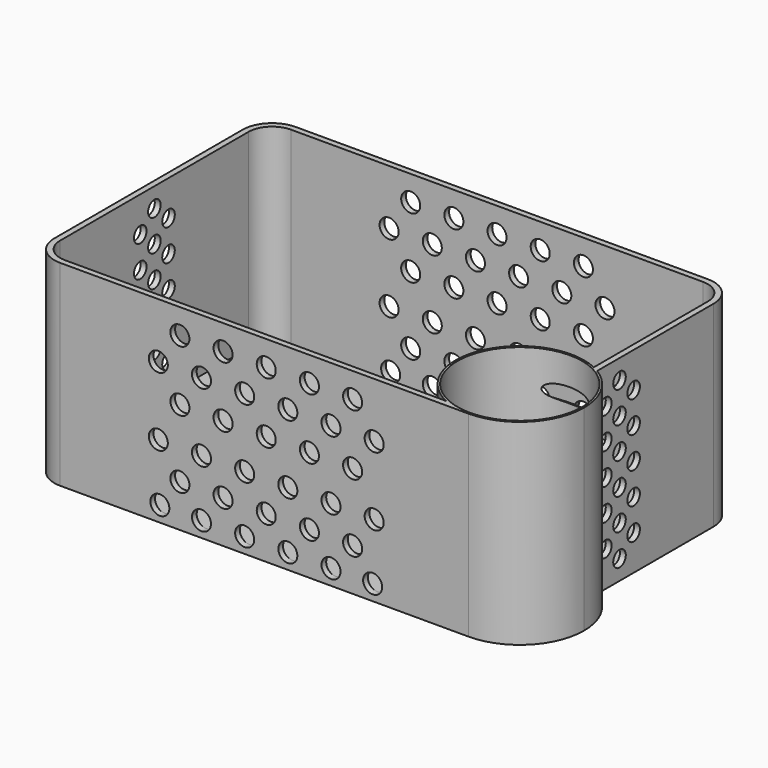
from build123d import *

# Parameters (mm, degrees)
F0_R     = 31.75
F1_DEPTH = 100
F3_DEPTH = 3
F5_D     = 9.7
F7_D     = 8


# Not quite as in the source:
# - a feature names something its author has since deleted; it is built from what else it names


with BuildPart() as f1:
    # F0 (on Top) → F1 (new body)
    with BuildSketch(Plane.XY):
        with BuildLine():
            Line((105, 75), (-105, 75))
            ThreePointArc((-105, 75), (-115.6066017178, 70.6066017178), (-120, 60))
            Line((-120, 60), (-120, -60))
            ThreePointArc((-120, -60), (-115.6066017178, -70.6066017178), (-105, -75))
            Line((-105, -75), (103, -75))
            ThreePointArc((103, -75), (95.9910771156, -74.2412097302), (89.3069360624, -72))
            Line((89.3069360624, -72), (-105, -72))
            ThreePointArc((-105, -72), (-113.4852813742, -68.4852813742), (-117, -60))
            Line((-117, -60), (-117, 60))
            ThreePointArc((-117, 60), (-113.4852813742, 68.4852813742), (-105, 72))
            Line((-105, 72), (105, 72))
            ThreePointArc((105, 72), (113.4852813742, 68.4852813742), (117, 60))
            Line((117, 60), (117, -12.6432017942))
            ThreePointArc((117, -12.6432017942), (118.5210097227, -13.4114709601), (120, -14.2578135902))
            Line((120, -14.2578135902), (120, 60))
            ThreePointArc((120, 60), (115.6066017178, 70.6066017178), (105, 75))
        make_face()
        with BuildLine():
            ThreePointArc((135.75, -42.25), (131.5421836936, -26.190540171), (120, -14.2578135902))
            ThreePointArc((120, -14.2578135902), (118.5210097227, -13.4114709601), (117, -12.6432017942))
            ThreePointArc((117, -12.6432017942), (73.3212041055, -28.4032829071), (89.3069360624, -72))
            ThreePointArc((89.3069360624, -72), (95.9910771156, -74.2412097302), (103, -75))
            ThreePointArc((103, -75), (126.1577470839, -65.4077470839), (135.75, -42.25))
        make_face()
        with Locations((103, -42.25)):
            Circle(F0_R, mode=Mode.SUBTRACT)
    extrude(amount=F1_DEPTH)

    # F2 (on Top) → F3 (join)
    with BuildSketch(Plane.XY):
        with BuildLine():
            ThreePointArc((117, -62), (114.0710678119, -69.0710678119), (107, -72))
            Line((107, -72), (89.3069360624, -72))
            ThreePointArc((89.3069360624, -72), (120.6651444382, -69.827258239), (135.75, -42.25))
            ThreePointArc((135.75, -42.25), (130.6682353973, -24.7276927889), (117, -12.6432017942))
            Line((117, -12.6432017942), (117, -62))
        make_face()
        with BuildLine():
            Line((89.3069360624, -72), (107, -72))
            ThreePointArc((107, -72), (114.0710678119, -69.0710678119), (117, -62))
            Line((117, -62), (117, -12.6432017942))
            ThreePointArc((117, -12.6432017942), (73.3212041055, -28.4032829071), (89.3069360624, -72))
        make_face()
        with BuildLine():
            Line((-107, -72), (89.3069360624, -72))
            ThreePointArc((89.3069360624, -72), (73.3212041055, -28.4032829071), (117, -12.6432017942))
            Line((117, -12.6432017942), (117, 62))
            ThreePointArc((117, 62), (114.0710678119, 69.0710678119), (107, 72))
            Line((107, 72), (-107, 72))
            ThreePointArc((-107, 72), (-114.0710678119, 69.0710678119), (-117, 62))
            Line((-117, 62), (-117, -62))
            ThreePointArc((-117, -62), (-114.0710678119, -69.0710678119), (-107, -72))
        make_face()
    extrude(amount=F3_DEPTH)

    # F5 (through all)
    with Locations(Plane.XZ.offset(75)):
        with Locations((-44, 87.2559348033), (-55, 71.9345058483), (-33, 71.9345058483), (-22, 87.2559348033), (-11, 71.9345058483), (0, 87.2559348033), (11, 71.9345058483), (22, 87.2559348033), (33, 71.9345058483), (44, 87.2559348033), (55, 71.9345058483), (55.0000035802, 36.9702333042), (44, 56.2202288289), (33, 36.9702333042), (22, 56.2202288289), (11, 36.9702333042), (0, 56.2202288289), (-11, 36.9702333042), (-33, 36.9702333042), (-22, 56.2202288289), (-44, 56.2202288289), (-55.0000035802, 36.9702333042), (-54.2142895502, 7.8988097195), (-44, 21.6488079294), (-33, 7.8988097195), (-22, 21.6488079294), (-11, 7.8988097195), (0, 21.6488079294), (11, 7.8988097195), (22, 21.6488079294), (33, 7.8988097195), (44, 21.6488079294), (54.2142895502, 7.8988097195)):
            Hole(F5_D / 2)

    # F7 (through all)
    with Locations(Plane.YZ.offset(120)):
        with Locations((0, 90), (0, 74), (0, 58), (9, 50), (-9, 50), (0, 42), (0, 26), (0, 10), (-9, 82), (-9, 66), (-9, 34), (-9, 18), (9, 82), (9, 66), (9, 34), (9, 18)):
            Hole(F7_D / 2)


solid = f1.part
